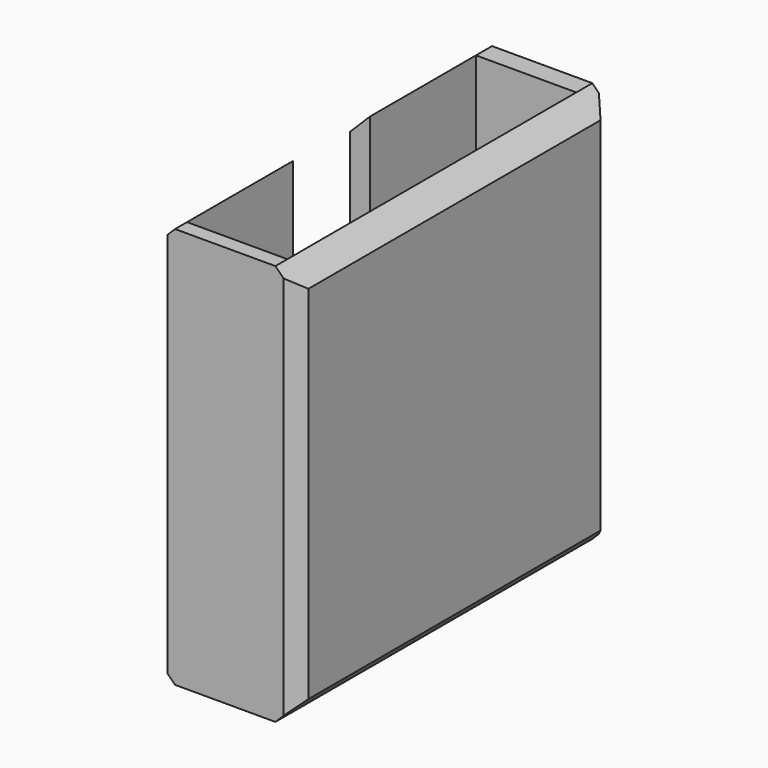
from build123d import *

# Parameters (mm, degrees)
F0_W     = 5
F0_H     = 18
F1_DEPTH = 20
F2_SIZE  = 0.99999
F3_W     = 4.7912499867
F3_H     = 21.5901492629
F4_DEPTH = 5


# Not quite as in the source:
# - a fillet or chamfer is up to 0.001 mm smaller than in the source, because OpenCascade refuses the exact size


with BuildPart() as f1:
    # F0 (on Top) → F1 (new body)
    with BuildSketch(Plane.XY):
        Polygon((-2.3178061422, 7.6096997074), (-7.9299724714, 7.6096997074), (-8.6440549978, 6.9096381776), (-8.6440549978, -11.3519806733), (-8.0234205974, -12.1360807569), (-2.2334722516, -12.1360807569), (-1.6440549978, -11.3282519997), (-1.6440549978, 6.8707413895), align=None)
        with Locations((-5.1440549978, -2.3903002926)):
            Rectangle(F0_W, F0_H, mode=Mode.SUBTRACT)
    extrude(amount=F1_DEPTH)

    # F2 (size 1 in the source; OpenCascade refuses exactly that, so slightly less here)
    f2_edges = [f1.edges().sort_by_distance(p)[0] for p in [
        (-8.644055, -2.221171, 20),
        (-8.644055, -2.221171, 0),
        (-1.644055, -2.228755, 0),
        (-1.644055, -2.228755, 20),
    ]]
    chamfer(f2_edges, length=F2_SIZE)

    # F3 (on face) → F4 (cut)
    with BuildSketch(Plane(origin=(-8.6440549978, 0, 0), x_dir=(0, -1, 0), z_dir=(-1, 0, 0))):
        with Locations((2.3956249934, 9.8618984921)):
            Rectangle(F3_W, F3_H)
    extrude(amount=-F4_DEPTH, mode=Mode.SUBTRACT)


solid = f1.part
